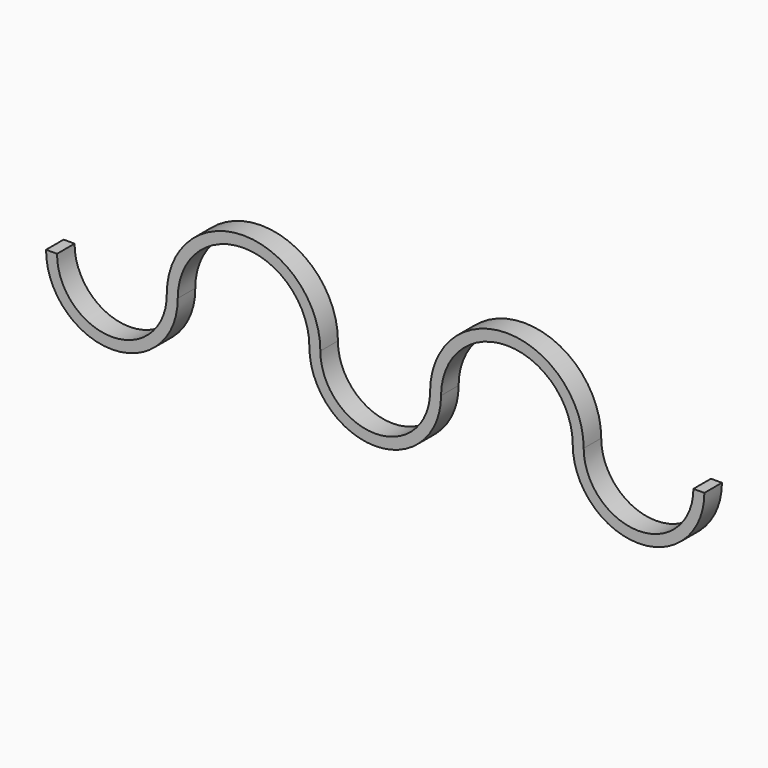
from build123d import *

# Parameters (mm, degrees)
F1_DEPTH = 5


# Not quite as in the source:
# - ends of sketch curves that miss each other by under 0.0002 mm in the source are joined


with BuildPart() as f1:
    # F0 (on Front) → F1 (new body)
    with BuildSketch(Plane.XZ):
        with BuildLine():
            Line((-8.2946076301, 0), (-10.7946076301, 0))
            ThreePointArc((-10.7946076301, 0), (4.2053923699, -15), (19.2053923699, 0))
            Line((19.2053923699, 0), (16.705392798, 0.0014630326))
            ThreePointArc((16.705392798, 0.0014630326), (4.2061241002, -12.4992684623), (-8.2946076301, 0))
        make_face()
        with BuildLine():
            ThreePointArc((-40.7946076301, 0), (-25.7946076301, 15), (-10.7946076301, 0))
            Line((-10.7946076301, 0), (-8.2946076301, 0))
            ThreePointArc((-8.2946076301, 0), (-25.7946076301, 17.5), (-43.2946076301, 0))
            Line((-43.2946076301, 0), (-40.7946076301, 0))
        make_face()
        with BuildLine():
            ThreePointArc((-70.7936146824, 0), (-55.7941111563, -15.1220408499), (-40.7946076301, 0))
            Line((-40.7946076301, 0), (-43.2946076301, 0))
            ThreePointArc((-43.2946076301, 0), (-55.7941111563, -12.6114073597), (-68.2936146824, 0))
            Line((-68.2936146824, 0), (-70.7936146824, 0))
        make_face()
        with BuildLine():
            Line((16.705392798, 0.0014630326), (19.2053923699, 0))
            ThreePointArc((19.2053923699, 0), (34.2052637046, 14.9378715725), (49.2051350393, 0))
            Line((49.2051350393, 0), (51.7051350393, 0))
            ThreePointArc((51.7051350393, 0), (34.205992633, 17.4335732975), (16.705392798, 0.0014630326))
        make_face()
        with BuildLine():
            Line((51.7051350393, 0), (49.2051350393, 0))
            ThreePointArc((49.2051350393, 0), (50.4551350393, -0.0521740711), (51.7051350393, 0))
        make_face()
        with BuildLine():
            ThreePointArc((51.7051350393, 0), (50.4551350393, -0.0521740711), (49.2051350393, 0))
            ThreePointArc((49.2051350393, 0), (64.205134968, -14.9985369674), (79.2051348966, 0))
            Line((79.2051348966, 0), (76.7051348966, 0))
            ThreePointArc((76.705134968, 0), (64.205134968, -12.5), (51.705134968, 0))
        make_face()
    extrude(amount=F1_DEPTH)


solid = f1.part
